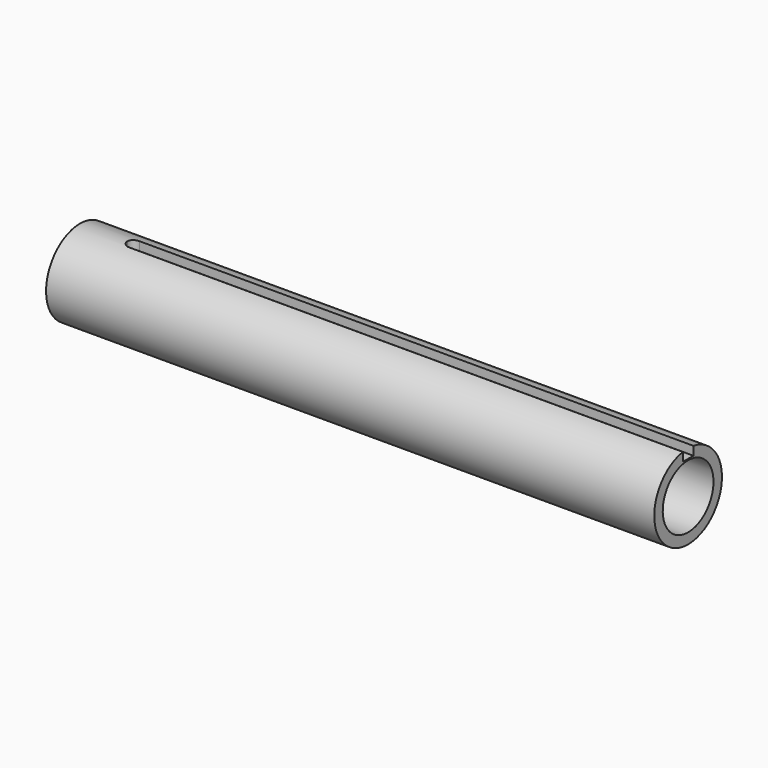
from build123d import *

# Parameters (mm, degrees)
F2_W     = 5
F2_H     = 4
F3_DEPTH = 212
F4_R     = 2.49999


# Not quite as in the source:
# - a fillet or chamfer is up to 0.001 mm smaller than in the source, because OpenCascade refuses the exact size
# - a feature names something its author has since deleted; it is built from what else it names


with BuildPart() as f1:
    # F0 (on Front) → F1 (revolve)
    with BuildSketch(Plane.XZ):
        Polygon((0, 12), (0, 16), (-230, 16), (-230, 11.9125), (-149.8207171315, 9.9), (-25, 9.9), (-25, 12), align=None)
    revolve(axis=Axis((-16.2521931838, 0, 0), (-1, 0, 0)))

    # F2 (on Right) → F3 (cut)
    with BuildSketch(Plane.YZ):
        with Locations((0, 14.5)):
            Rectangle(F2_W, F2_H)
    extrude(amount=-F3_DEPTH, mode=Mode.SUBTRACT)

    # F4 (radius 2.5 in the source; OpenCascade refuses exactly that, so slightly less here)
    f4_edges = [f1.edges().sort_by_distance(p)[0] for p in [
        (-212, 2.5, 14.15174),
        (-212, -2.5, 14.15174),
    ]]
    fillet(f4_edges, radius=F4_R)


solid = f1.part
